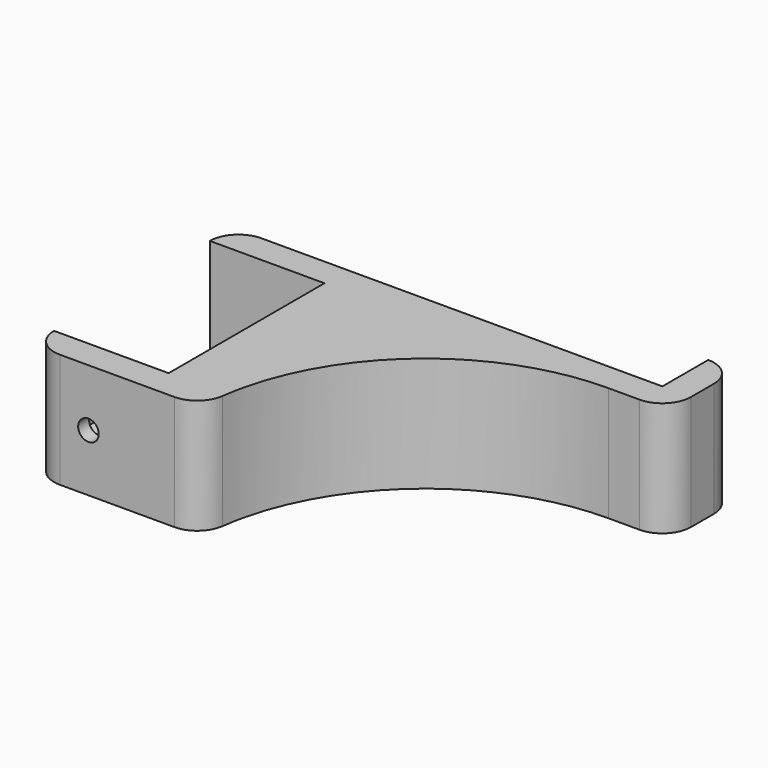
from build123d import *

# Parameters (mm, degrees)
F3_DEPTH = 20
F4_R     = 4.99999
F6_DEPTH = 2.6
F7_D     = 3.6
F7_DEPTH = 10
F7_TIP   = 1.0815491142
F8_R     = 40


# Not quite as in the source:
# - a fillet or chamfer is up to 0.001 mm smaller than in the source, because OpenCascade refuses the exact size


with BuildPart() as f3:
    # F2 (on Top) → F3 (new body)
    with BuildSketch(Plane.XY):
        Polygon((0, 5), (0, 0), (20, 0), (20, -34), (0, -34), (0, -39), (30, -39), (30, 0), (80, 0), (80, 15), (75, 15), (75, 5), align=None)
    extrude(amount=F3_DEPTH)

    # F4 (radius 5 in the source; OpenCascade refuses exactly that, so slightly less here)
    f4_edges = [f3.edges().sort_by_distance(p)[0] for p in [
        (30, -39, 10),
        (80, 0, 10),
        (80, 15, 10),
        (0, 5, 10),
        (0, -39, 10),
    ]]
    fillet(f4_edges, radius=F4_R)

    # F5 (on face) → F6 (cut)
    with BuildSketch(Plane(origin=(0, -34, 0), x_dir=(-1, 0, 0), z_dir=(0, 1, 0))):
        Polygon((-7.25, 8.4122867597), (-7.25, 11.5877132403), (-10, 13.1754264805), (-12.75, 11.5877132403), (-12.75, 8.4122867597), (-10, 6.8245735195), align=None)
    extrude(amount=-F6_DEPTH, mode=Mode.SUBTRACT)

    # F7 (one way)
    with BuildSketch(Plane(origin=(0, -34, 0), x_dir=(-1, 0, 0), z_dir=(0, 1, 0))):
        with Locations((-10, 10)):
            Circle(F7_D / 2)
    extrude(amount=-F7_DEPTH, mode=Mode.SUBTRACT)
    with Locations(Plane(origin=(0, -34, 0), x_dir=(-1, 0, 0), z_dir=(0, 1, 0))):
        with Locations((-10, 10)):
            with Locations((0, 0, -(F7_DEPTH + F7_TIP / 2))):  # 118° drill point
                Cone(0, F7_D / 2, F7_TIP, mode=Mode.SUBTRACT)

    # F8
    f8_edges = [f3.edges().sort_by_distance(p)[0] for p in [
        (30, 0, 10),
    ]]
    fillet(f8_edges, radius=F8_R)


solid = f3.part
